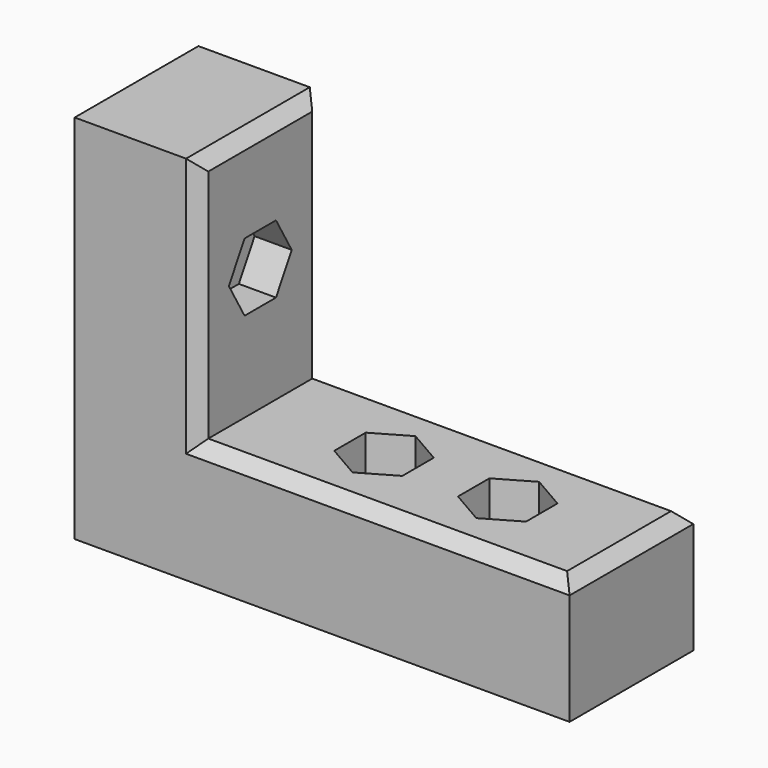
from build123d import *

# Parameters (mm, degrees)
F0_W     = 30
F0_H     = 12.5
F0_R     = 1.55
F1_DEPTH = 10
F0_W_2   = 10
F2_DEPTH = 30
F3_R     = 1.55
F4_DEPTH = 10
F5_SIZE  = 1
F7_DEPTH = 3
F9_DEPTH = 3


# Not quite as in the source:
# - a feature names something its author has since deleted; it is built from what else it names


with BuildPart() as f1:
    # F0 (on Top) → F1 (new body)
    with BuildSketch(Plane.XY):
        with Locations((25, 6.25)):
            Rectangle(F0_W, F0_H)
        with Locations((20, 6.25)):
            Circle(F0_R, mode=Mode.SUBTRACT)
        with Locations((30, 6.25)):
            Circle(F0_R, mode=Mode.SUBTRACT)
    extrude(amount=F1_DEPTH)

    # F0 (on Top) → F2 (join)
    with BuildSketch(Plane.XY):
        with Locations((5, 6.25)):
            Rectangle(F0_W_2, F0_H)
    extrude(amount=F2_DEPTH)

    # F3 (on face) → F4 (cut)
    with BuildSketch(Plane(origin=(0, 0, 0), x_dir=(0, -1, 0), z_dir=(-1, 0, 0))):
        with Locations((-6.25, 20)):
            Circle(F3_R)
    extrude(amount=-F4_DEPTH, mode=Mode.SUBTRACT)

    # F5
    f5_edges = [f1.edges().sort_by_distance(p)[0] for p in [
        (25, 0, 10),
        (40, 6.25, 10),
        (25, 12.5, 10),
        (10, 12.5, 20),
        (10, 6.25, 30),
        (10, 0, 20),
    ]]
    chamfer(f5_edges, length=F5_SIZE)

    # F6 (on face) → F7 (cut)
    with BuildSketch(Plane.XY.offset(10)):
        Polygon((22.75, 4.6622867597), (22.75, 7.8377132403), (20, 9.4254264805), (17.25, 7.8377132403), (17.25, 4.6622867597), (20, 3.0745735195), align=None)
        Polygon((32.75, 4.6622867597), (32.75, 7.8377132403), (30, 9.4254264805), (27.25, 7.8377132403), (27.25, 4.6622867597), (30, 3.0745735195), align=None)
    extrude(amount=-F7_DEPTH, mode=Mode.SUBTRACT)

    # F8 (on face) → F9 (cut)
    with BuildSketch(Plane.YZ.offset(10)):
        Polygon((4.6622867597, 17.25), (7.8377132403, 17.25), (9.4254264805, 20), (7.8377132403, 22.75), (4.6622867597, 22.75), (3.0745735195, 20), align=None)
    extrude(amount=-F9_DEPTH, mode=Mode.SUBTRACT)


solid = f1.part
